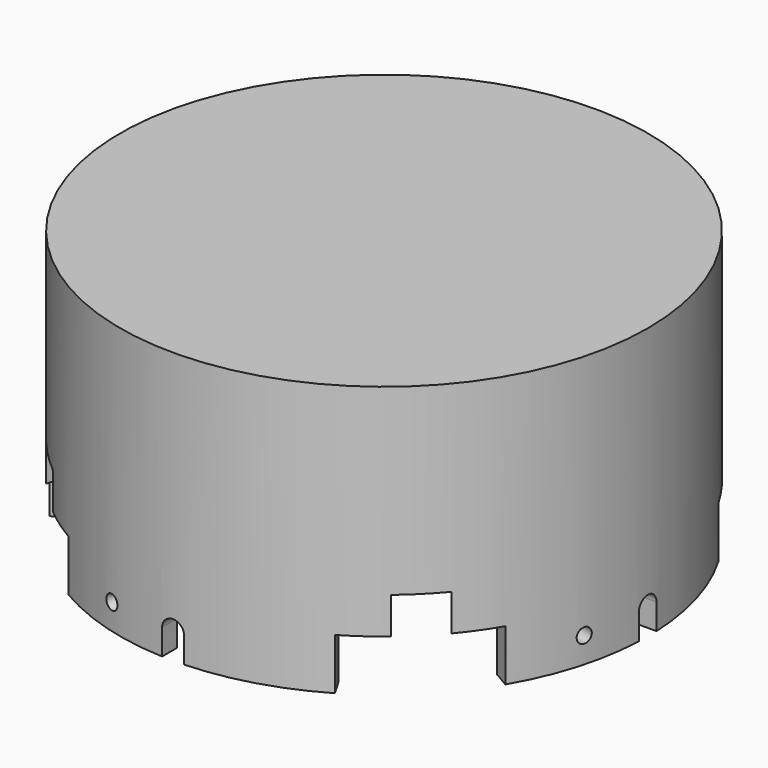
from build123d import *

# Parameters (mm, degrees)
F0_R             = 36
F1_DEPTH         = 37
F2_T             = -2.5
F4_DEPTH         = 7
F4_COPIES_COUNT  = 4
F5_R             = 4
F6_DEPTH         = 12
F6_COPIES_COUNT  = 4
F10_D            = 2
F10_DEPTH        = 10
F10_START        = 0.1138917
F10_TIP          = 0.600860619
F10_COPIES_COUNT = 4
F14_DEPTH        = 5
F14_COPIES_COUNT = 4


# Not quite as in the source:
# - a pattern or mirror of a feature is missing from the dataset's text; its kind, count and spacing are read off the source's solid


with BuildPart() as f1:
    # F0 (on Top) → F1 (new body)
    with BuildSketch(Plane.XY):
        Circle(F0_R)
    extrude(amount=F1_DEPTH)

    # F2
    f2_openings = [f1.faces().sort_by_distance(p)[0] for p in [
        (0, 0, 0),
    ]]
    offset(amount=F2_T, openings=f2_openings)

    # F3 (on Top) → F4 (cut)
    with BuildSketch(Plane.XY):
        with BuildLine():
            Line((31.0817403025, -18.1638492552), (28.9232861149, -16.9024708347))
            ThreePointArc((28.9232861149, -16.9024708347), (23.6880771697, -23.6880771697), (16.9024708347, -28.9232861149))
            Line((16.9024708347, -28.9232861149), (18.1638492552, -31.0817403025))
            ThreePointArc((18.1638492552, -31.0817403025), (25.4558441227, -25.4558441227), (31.0817403025, -18.1638492552))
        make_face()
    f4 = extrude(amount=F4_DEPTH, mode=Mode.SUBTRACT)

    # F4_copies: F4 ×4 about axis
    f4_copies_axis = Axis((0, 0, 0), (0, 0, 1))
    for i in range(1, F4_COPIES_COUNT):
        add(f4.rotate(f4_copies_axis, i * 360 / F4_COPIES_COUNT), mode=Mode.SUBTRACT)

    # F5 (on Top) → F6 (cut)
    with BuildSketch(Plane.XY):
        with Locations((23.6880771697, -23.6880771697)):
            Circle(F5_R)
    f6 = extrude(amount=F6_DEPTH, mode=Mode.SUBTRACT)

    # F6_copies: F6 ×4 about axis
    f6_copies_axis = Axis((0, 0, 0), (0, 0, 1))
    for i in range(1, F6_COPIES_COUNT):
        add(f6.rotate(f6_copies_axis, i * 360 / F6_COPIES_COUNT), mode=Mode.SUBTRACT)

    # F10
    # its depths count from where the whole tool has entered the part; down to there all is cleared
    with Locations(Plane(origin=(-9.3433675282, -34.869922329, 0), x_dir=(0.9659258263, -0.2588190451, 0), z_dir=(-0.2588190451, -0.9659258263, 0)).offset(-F10_START)):
        with Locations((0, 3.5)):
            f10 = Hole(F10_D / 2, depth=F10_DEPTH)
            with Locations((0, 0, -(F10_DEPTH + F10_TIP / 2))):  # 118° drill point
                Cone(0, F10_D / 2, F10_TIP, mode=Mode.SUBTRACT)

    # F10_copies: F10 ×4 about axis
    f10_copies_axis = Axis((0, 0, 0), (0, 0, 1))
    for i in range(1, F10_COPIES_COUNT):
        add(f10.rotate(f10_copies_axis, i * 360 / F10_COPIES_COUNT), mode=Mode.SUBTRACT)

    # F13 (on line) → F14 (cut)
    with BuildSketch(Plane.XZ.offset(36)):
        with BuildLine():
            ThreePointArc((1.5, 3.5), (0, 5), (-1.5, 3.5))
            Line((-1.5, 3.5), (-1.5, 0))
            Line((-1.5, 0), (1.5, 0))
            Line((1.5, 0), (1.5, 3.5))
        make_face()
    f14 = extrude(amount=-F14_DEPTH, mode=Mode.SUBTRACT)

    # F14_copies: F14 ×4 about axis
    f14_copies_axis = Axis((0, 0, 0), (0, 0, 1))
    for i in range(1, F14_COPIES_COUNT):
        add(f14.rotate(f14_copies_axis, i * 360 / F14_COPIES_COUNT), mode=Mode.SUBTRACT)


solid = f1.part
